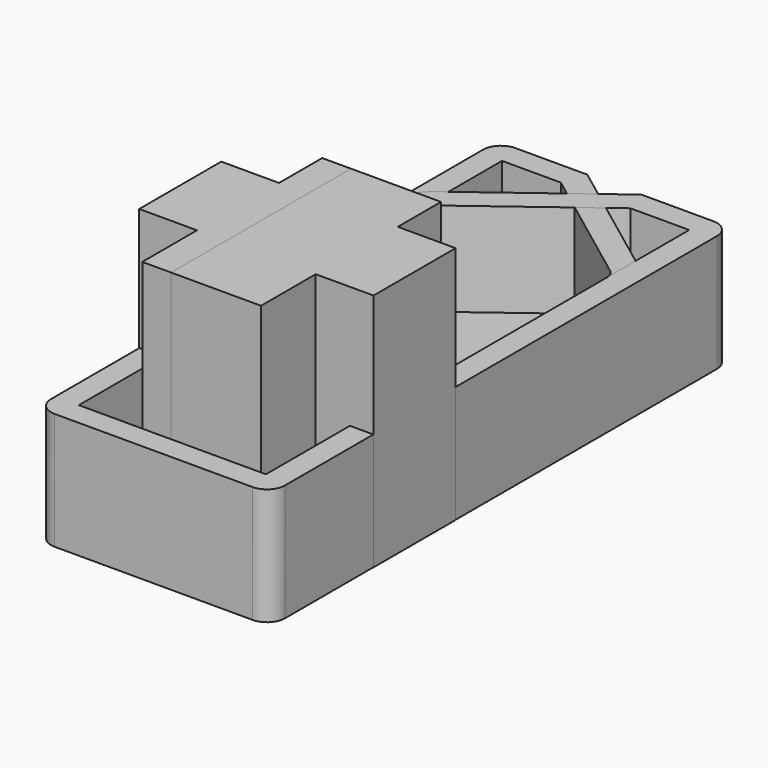
from build123d import *

# Parameters (mm, degrees)
F1_DEPTH = 6.5
F2_T     = -1.3
F4_DEPTH = 13.3


# Not quite as in the source:
# - a feature names something its author has since deleted; it is built from what else it names


with BuildPart() as f1:
    # F0 (on Top) → F1 (new body)
    with BuildSketch(Plane.XY):
        with BuildLine():
            Line((-5.5, -13), (5.5, -13))
            ThreePointArc((5.5, -13), (6.2071067812, -12.7071067812), (6.5, -12))
            Line((6.5, -12), (6.5, 12))
            ThreePointArc((6.5, 12), (6.288854382, 12.894427191), (5.7, 13.6))
            Line((5.7, 13.6), (-1.5, 19))
            Line((-1.5, 19), (-5.5, 19))
            ThreePointArc((-5.5, 19), (-6.2071067812, 18.7071067812), (-6.5, 18))
            Line((-6.5, 18), (-6.5, 13))
            Line((-6.5, 13), (-6.5, -12))
            ThreePointArc((-6.5, -12), (-6.2071067812, -12.7071067812), (-5.5, -13))
        make_face()
    extrude(amount=F1_DEPTH)

    # F2
    f2_openings = [f1.faces().sort_by_distance(p)[0] for p in [
        (-0.234078, 2.146096, 6.5),
    ]]
    offset(amount=F2_T, openings=f2_openings)

    # F3 (on Top) → F4 (join)
    with BuildSketch(Plane.XY):
        Polygon((-3.3, -9.6670114048), (1.7, -9.6670114048), (1.7, 2.8329885952), (-3.3, 2.8329885952), (-3.3, -0.1670114048), (-6.5110628493, -0.1670114048), (-6.5110628493, -5.8670114048), (-3.3, -5.8670114048), align=None)
    extrude(amount=F4_DEPTH)


with BuildPart() as f6_1:
    # F6: instance of F1
    add(f1.part.mirror(Plane.YZ))


solid = Compound([f1.part, f6_1.part])
